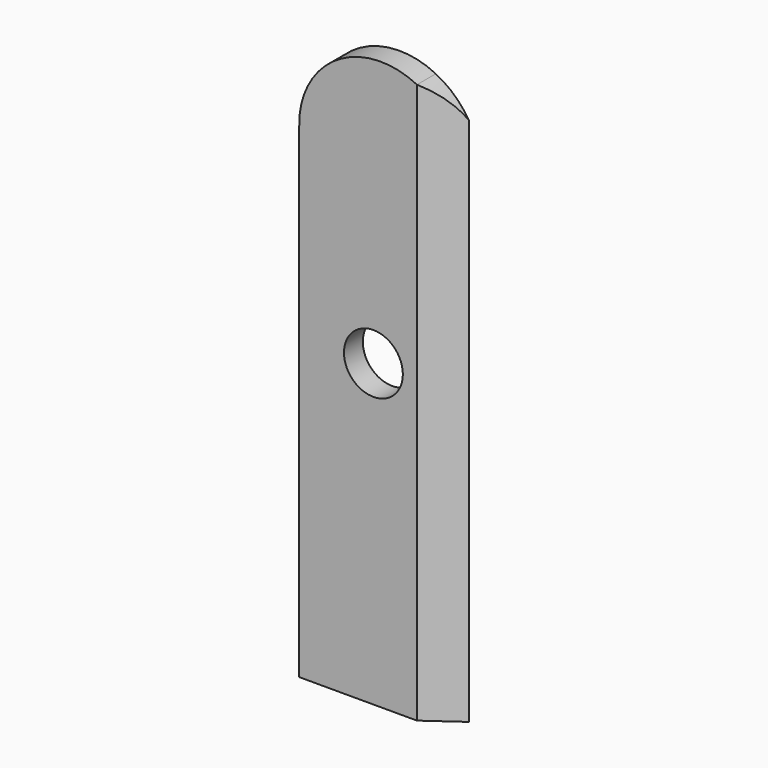
from build123d import *

# Parameters (mm, degrees)
F0_R     = 0.125
F1_DEPTH = 0.1
F2_SIZE2 = 0.09999
F2_SIZE  = 0.13999


# Not quite as in the source:
# - a fillet or chamfer is up to 0.001 mm smaller than in the source, because OpenCascade refuses the exact size


with BuildPart() as f1:
    # F0 (on Front) → F1 (new body)
    with BuildSketch(Plane.XZ):
        with BuildLine():
            Line((0, 2.06), (0, 0))
            Line((0, 0), (0.5, 0))
            Line((0.5, 0), (0.5, 2.3774036342))
            ThreePointArc((0.5, 2.3774036342), (0.1605070536, 2.3596783794), (0, 2.06))
        make_face()
        with Locations((0.315, 1.275)):
            Circle(F0_R, mode=Mode.SUBTRACT)
        with BuildLine():
            Line((0.5, 2.3774036342), (0.5, 0))
            Line((0.5, 0), (0.64, 0))
            Line((0.64, 0), (0.64, 2.25))
            ThreePointArc((0.64, 2.25), (0.5788806325, 2.3234604755), (0.5, 2.3774036342))
        make_face()
    extrude(amount=F1_DEPTH)

    # F2 (size 0.14 and 0.1 in the source; OpenCascade refuses exactly that, so slightly less here)
    f2_edges = [f1.edges().sort_by_distance(p)[0] for p in [
        (0.64, -0.1, 1.125),
    ]]
    f2_side = f1.faces().sort_by_distance((0.02497, -0.1, 1.03))[0]
    chamfer(f2_edges, length=F2_SIZE, length2=F2_SIZE2, reference=f2_side)


solid = f1.part
